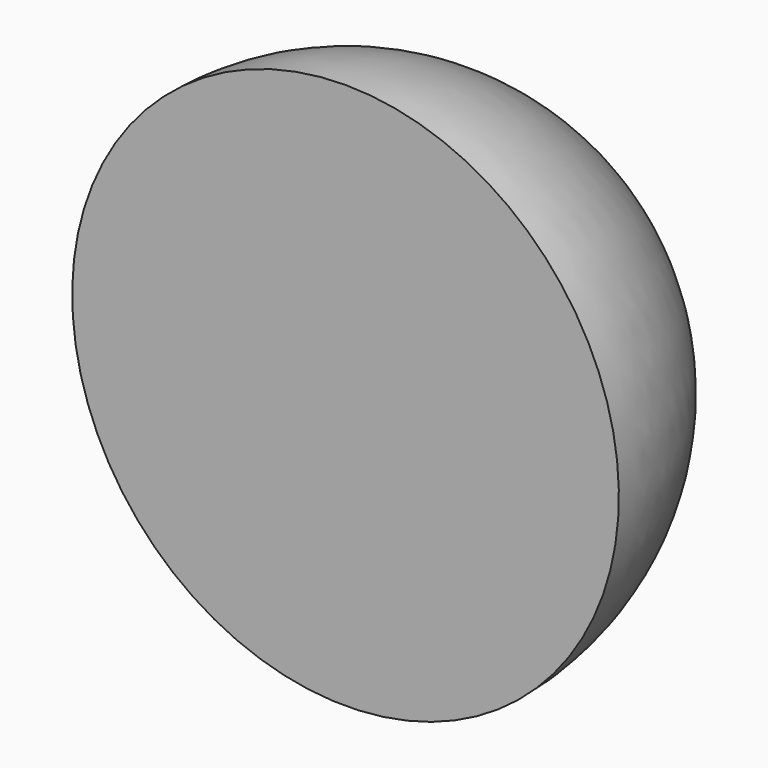
from build123d import *


# Not quite as in the source:
# - a feature names something its author has since deleted; it is built from what else it names


with BuildPart() as f1:
    # F0 (on Right) → F1 (revolve)
    with BuildSketch(Plane.YZ):
        with BuildLine():
            ThreePointArc((12.5812348626, 0), (8.7747298529, 8.6988771492), (0, 12.3271081309))
            Line((0, 12.3271081309), (0, 0))
            Line((0, 0), (12.5812348626, 0))
        make_face()
    revolve(axis=Axis((0, 6.2906174313, 0), (0, -1, 0)))


solid = f1.part
